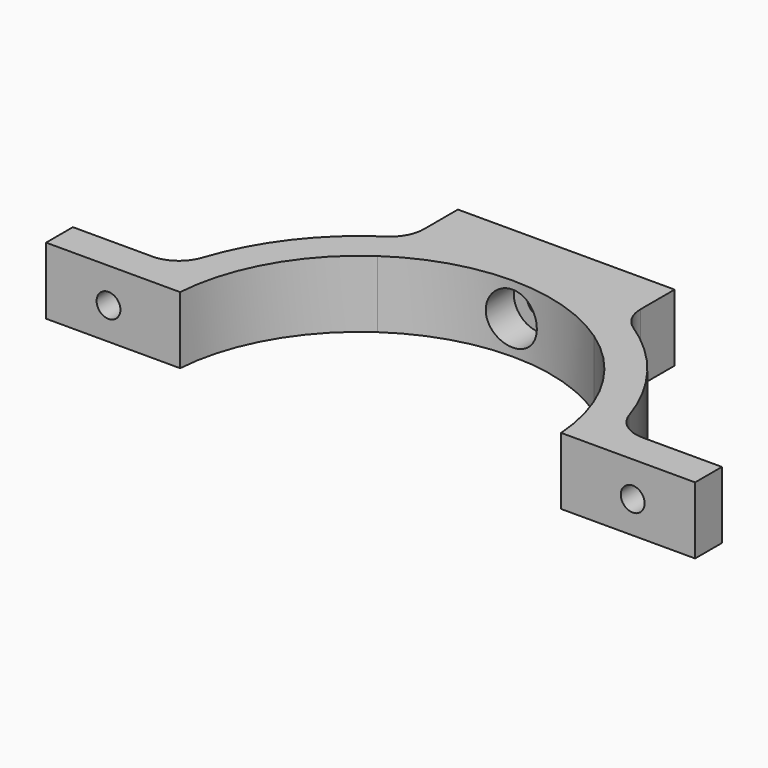
from build123d import *
from build123d import SkipClean  # not in build123d's __all__

# Parameters (mm, degrees)
F1_DEPTH       = 10
F3_D           = 3.556
F3_CBORE_D     = 7.62
F3_CBORE_DEPTH = 10
F4_DEPTH       = 10.001
F6_D           = 3.556
F7_R           = 5


# Not quite as in the source:
# - a feature names something its author has since deleted; it is built from what else it names


with BuildPart() as f1:
    # F0 (on Top) → F1 (new body)
    with BuildSketch(Plane.XY):
        with BuildLine():
            ThreePointArc((16.1705551086, 23.468343518), (24.7491207645, 14.1326225939), (28.4297379517, 2))
            Line((28.4297379517, 2), (28.4297379517, 7))
            Line((28.4297379517, 7), (32.7604945018, 7))
            ThreePointArc((32.7604945018, 7), (26.8945535829, 19.9733068763), (16.1705551086, 29.3387652685))
            Line((16.1705551086, 29.3387652685), (16.1705551086, 23.468343518))
        make_face()
        with BuildLine():
            ThreePointArc((-16.1705551086, 23.468343518), (0, 28.5), (16.1705551086, 23.468343518))
            Line((16.1705551086, 23.468343518), (16.1705551086, 29.3387652685))
            Line((16.1705551086, 29.3387652685), (-16.1705551086, 29.3387652685))
            Line((-16.1705551086, 29.3387652685), (-16.1705551086, 23.468343518))
        make_face()
        with BuildLine():
            ThreePointArc((-28.4297379517, 2), (-24.7491207645, 14.1326225939), (-16.1705551086, 23.468343518))
            Line((-16.1705551086, 23.468343518), (-16.1705551086, 29.3387652685))
            ThreePointArc((-16.1705551086, 29.3387652685), (-26.8945535829, 19.9733068763), (-32.7604945018, 7))
            Line((-32.7604945018, 7), (-28.4297379517, 7))
            Line((-28.4297379517, 7), (-28.4297379517, 2))
        make_face()
        with BuildLine():
            Line((-48.4297379517, 2), (-33.4402452144, 2))
            ThreePointArc((-33.4402452144, 2), (-33.1946454228, 4.5128167765), (-32.7604945018, 7))
            Line((-32.7604945018, 7), (-48.4297379517, 7))
            Line((-48.4297379517, 7), (-48.4297379517, 2))
        make_face()
        with BuildLine():
            Line((-33.4402452144, 2), (-28.4297379517, 2))
            Line((-28.4297379517, 2), (-28.4297379517, 7))
            Line((-28.4297379517, 7), (-32.7604945018, 7))
            ThreePointArc((-32.7604945018, 7), (-33.1946454228, 4.5128167765), (-33.4402452144, 2))
        make_face()
        with BuildLine():
            Line((28.4297379517, 7), (28.4297379517, 2))
            Line((28.4297379517, 2), (33.4402452144, 2))
            ThreePointArc((33.4402452144, 2), (33.1946454228, 4.5128167765), (32.7604945018, 7))
            Line((32.7604945018, 7), (28.4297379517, 7))
        make_face()
        with BuildLine():
            ThreePointArc((32.7604945018, 7), (33.1946454228, 4.5128167765), (33.4402452144, 2))
            Line((33.4402452144, 2), (48.4297379517, 2))
            Line((48.4297379517, 2), (48.4297379517, 7))
            Line((48.4297379517, 7), (32.7604945018, 7))
        make_face()
        with BuildLine():
            Line((-16.1705551086, 33.5), (-16.1705551086, 29.3387652685))
            ThreePointArc((-16.1705551086, 29.3387652685), (-8.3486933282, 32.4430165014), (1.811e-07, 33.5))
            Line((1.811e-07, 33.5), (-16.1705551086, 33.5))
        make_face()
        with BuildLine():
            ThreePointArc((1.811e-07, 33.5), (8.3486935036, 32.4430164563), (16.1705551086, 29.3387652685))
            Line((16.1705551086, 29.3387652685), (16.1705551086, 33.5))
            Line((16.1705551086, 33.5), (1.811e-07, 33.5))
        make_face()
        with BuildLine():
            Line((-16.1705551086, 23.468343518), (16.1705551086, 23.468343518))
            ThreePointArc((16.1705551086, 23.468343518), (0, 28.5), (-16.1705551086, 23.468343518))
        make_face()
        Polygon((-16.1705551086, 33.5), (1.811e-07, 33.5), (16.1705551086, 33.5), (16.1705551086, 38.5), (-16.1705551086, 38.5), align=None)
        with BuildLine():
            Line((-16.1705551086, 29.3387652685), (16.1705551086, 29.3387652685))
            ThreePointArc((16.1705551086, 29.3387652685), (8.3486935036, 32.4430164563), (1.811e-07, 33.5))
            ThreePointArc((1.811e-07, 33.5), (-8.3486933282, 32.4430165014), (-16.1705551086, 29.3387652685))
        make_face()
    extrude(amount=F1_DEPTH)

    # F3 (through all)
    with Locations(Plane.XZ.offset(-23.468343518)):
        with Locations((0, 5)):
            CounterBoreHole(F3_D / 2, F3_CBORE_D / 2, F3_CBORE_DEPTH)

    # F0 (on Top) → F4 (cut, through all)
    with BuildSketch(Plane.XY):
        with BuildLine():
            Line((-16.1705551086, 23.468343518), (16.1705551086, 23.468343518))
            ThreePointArc((16.1705551086, 23.468343518), (0, 28.5), (-16.1705551086, 23.468343518))
        make_face()
    with SkipClean():  # cleaning this boolean's faces spoils the solid; the shape is the same uncleaned
        extrude(amount=F4_DEPTH, mode=Mode.SUBTRACT)

    # F6 (through all)
    with Locations(Plane.XZ.offset(-2)):
        with Locations((-39.116, 4.78035165), (39.116, 4.78035165)):
            Hole(F6_D / 2)

    # F7
    f7_edges = [f1.edges().sort_by_distance(p)[0] for p in [
        (-32.760495, 7, 5),
        (32.760495, 7, 5),
        (16.170555, 29.338765, 5),
        (-16.170555, 29.338765, 5),
    ]]
    fillet(f7_edges, radius=F7_R)


solid = f1.part
